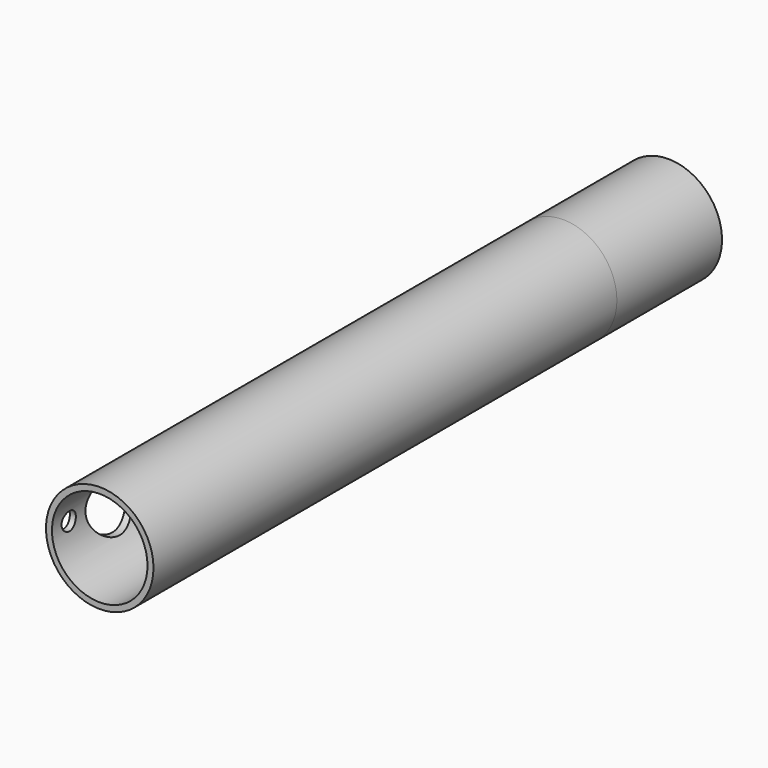
from build123d import *

# Parameters (mm, degrees)
F3_R      = 4.5
F4_DEPTH  = 39.5
F8_DEPTH  = 39.5
F6_R      = 4.5
F6_R_2    = 4
F9_DEPTH  = 9
F7_R      = 4.5
F7_R_2    = 4
F10_DEPTH = 11
F11_R     = 2.5
F11_R_2   = 0.75
F12_DEPTH = 4.501


# Not quite as in the source:
# - ends of sketch curves that miss each other by under 0.0002 mm in the source are joined


with BuildPart() as f4:
    # F3 (on Front) → F4 (new body)
    with BuildSketch(Plane.XZ):
        Circle(F3_R)
    extrude(amount=F4_DEPTH)

    # F5 (on face) → F8 (cut, through all)
    with BuildSketch(Plane.XZ.offset(39.5)):
        with BuildLine():
            Line((-1.25, -3.8), (0, -3.8))
            Line((0, -3.8), (1.25, -3.8))
            Line((1.25, -3.8), (1.25, -3.7))
            ThreePointArc((1.25, -3.7), (1.3085786438, -3.5585786438), (1.45, -3.5))
            Line((1.45, -3.5), (2, -3.5))
            Line((2, -3.5), (2, -3.05))
            ThreePointArc((2, -3.05), (2.0585786438, -2.9085786438), (2.2, -2.85))
            Line((2.2, -2.85), (3.15, -2.85))
            Line((3.15, -2.85), (3.15, -2.15))
            Line((3.15, -2.15), (2.2, -2.15))
            ThreePointArc((2.2, -2.15), (2.0585786438, -2.0914213562), (2, -1.95))
            Line((2, -1.95), (2, -1.887459))
            ThreePointArc((2, -1.887459), (2.1033535752, -1.771554046), (2.2, -1.65))
            Line((2.2, -1.65), (3.75, -1.65))
            Line((3.75, -1.65), (3.75, 0))
            Line((3.75, 0), (3.75, 1.65))
            Line((3.75, 1.65), (2.2, 1.65))
            ThreePointArc((2.2, 1.65), (2.1033535752, 1.771554046), (1.9999998047, 1.8874588157))
            Line((1.9999998047, 1.8874588157), (2, 1.95))
            ThreePointArc((2, 1.95), (2.0585786438, 2.0914213562), (2.2, 2.15))
            Line((2.2, 2.15), (3.15, 2.15))
            Line((3.15, 2.15), (3.15, 2.85))
            Line((3.15, 2.85), (2.2, 2.85))
            ThreePointArc((2.2, 2.85), (2.0585786438, 2.9085786438), (2, 3.05))
            Line((2, 3.05), (2, 3.5))
            Line((2, 3.5), (1.45, 3.5))
            ThreePointArc((1.45, 3.5), (1.3085786438, 3.5585786438), (1.25, 3.7))
            Line((1.25, 3.7), (1.25, 3.8))
            Line((1.25, 3.8), (0, 3.8))
            Line((0, 3.8), (-1.25, 3.8))
            Line((-1.25, 3.8), (-1.25, 3.7))
            ThreePointArc((-1.25, 3.7), (-1.3085786438, 3.5585786438), (-1.45, 3.5))
            Line((-1.45, 3.5), (-2, 3.5))
            Line((-2, 3.5), (-2, 3.05))
            ThreePointArc((-2, 3.05), (-2.0585786438, 2.9085786438), (-2.2, 2.85))
            Line((-2.2, 2.85), (-3.15, 2.85))
            Line((-3.15, 2.85), (-3.15, 2.15))
            Line((-3.15, 2.15), (-2.2, 2.15))
            ThreePointArc((-2.2, 2.15), (-2.0585786438, 2.0914213562), (-2, 1.95))
            Line((-2, 1.95), (-2, 1.887459))
            ThreePointArc((-2, 1.887459), (-2.1033535752, 1.771554046), (-2.2, 1.65))
            Line((-2.2, 1.65), (-3.75, 1.65))
            Line((-3.75, 1.65), (-3.75, 0))
            Line((-3.75, 0), (-3.75, -1.65))
            Line((-3.75, -1.65), (-2.2, -1.65))
            ThreePointArc((-2.2, -1.65), (-2.1033535752, -1.771554046), (-1.9999998047, -1.8874588157))
            Line((-1.9999998047, -1.8874588157), (-2, -1.95))
            ThreePointArc((-2, -1.95), (-2.0585786438, -2.0914213562), (-2.2, -2.15))
            Line((-2.2, -2.15), (-3.15, -2.15))
            Line((-3.15, -2.15), (-3.15, -2.85))
            Line((-3.15, -2.85), (-2.2, -2.85))
            ThreePointArc((-2.2, -2.85), (-2.0585786438, -2.9085786438), (-2, -3.05))
            Line((-2, -3.05), (-2, -3.5))
            Line((-2, -3.5), (-1.45, -3.5))
            ThreePointArc((-1.45, -3.5), (-1.3085786438, -3.5585786438), (-1.25, -3.7))
            Line((-1.25, -3.7), (-1.25, -3.8))
        make_face()
    extrude(amount=-F8_DEPTH, mode=Mode.SUBTRACT)

    # F6 (on face) → F9 (join)
    with BuildSketch(Plane.XZ.offset(39.5)):
        Circle(F6_R)
        Circle(F6_R_2, mode=Mode.SUBTRACT)
    extrude(amount=F9_DEPTH)

    # F7 (on face) → F10 (join)
    with BuildSketch(Plane(origin=(0, 0, 0), x_dir=(-1, 0, 0), z_dir=(0, 1, 0))):
        Circle(F7_R)
        Circle(F7_R_2, mode=Mode.SUBTRACT)
    extrude(amount=F10_DEPTH)

    # F11 (on Right) → F12 (cut, through all)
    with BuildSketch(Plane.YZ):
        with Locations((-42.5, 0)):
            Circle(F11_R)
        with Locations((-46.75, 0)):
            Circle(F11_R_2)
    extrude(amount=-F12_DEPTH, mode=Mode.SUBTRACT)


solid = f4.part
